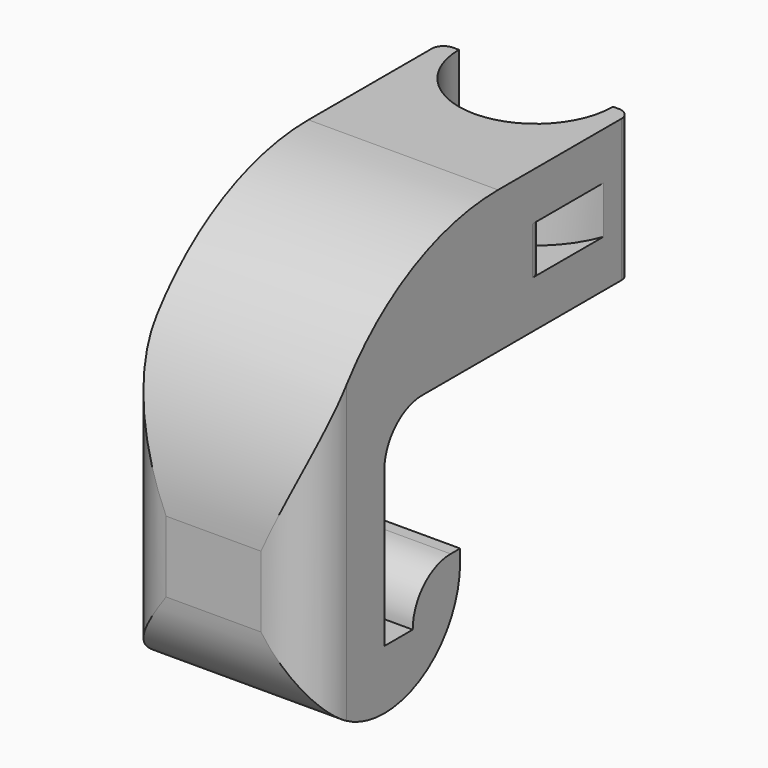
from build123d import *

# Parameters (mm, degrees)
F1_DEPTH     = 16
F2_R         = 7.99999
F3_R         = 20
F4_R         = 3.99999
F6_DEPTH     = 34.001
F8_DEPTH     = 4
F11_R        = 1
F12_T1_DEPTH = 33.00001


# Not quite as in the source:
# - a fillet or chamfer that OpenCascade refuses, or shapes differently, is made with other operations: its cross-section is extruded or revolved along the edge and cut away or added
# - a fillet or chamfer is up to 0.001 mm smaller than in the source, because OpenCascade refuses the exact size


with BuildPart() as f1:
    # F0 (on Right) → F1 (new body)
    with BuildSketch(Plane.YZ):
        Polygon((34, 34), (0, 34), (0, 0), (16, 0), (16, 9), (11, 9), (11, 5), (8, 5), (8, 22), (34, 22), align=None)
    extrude(amount=F1_DEPTH)

    # F2 (radius 8 in the source; OpenCascade refuses exactly that, so slightly less here)
    f2_edges = [f1.edges().sort_by_distance(p)[0] for p in [
        (8, 16, 0),
        (8, 0, 0),
    ]]
    fillet(f2_edges, radius=F2_R)

    # F3
    f3_edges = [f1.edges().sort_by_distance(p)[0] for p in [
        (8, 0, 34),
    ]]
    fillet(f3_edges, radius=F3_R)

    # F4 (radius 4 in the source; OpenCascade refuses exactly that, so slightly less here)
    f4_edges = [f1.edges().sort_by_distance(p)[0] for p in [
        (8, 8, 22),
        (8, 11, 9),
    ]]
    fillet(f4_edges, radius=F4_R)

    # F5 (on face) → F6 (cut, through all)
    with BuildSketch(Plane.XY.offset(34)):
        with BuildLine():
            ThreePointArc((1.5, 34), (8, 27.5), (14.5, 34))
            Line((14.5, 34), (1.5, 34))
        make_face()
    extrude(amount=-F6_DEPTH, mode=Mode.SUBTRACT)


with BuildPart() as f8:
    # F7 (on face) → F8 (new body)
    with BuildSketch(Plane.XY.offset(34)):
        with BuildLine():
            ThreePointArc((16, 31.1277186767), (8, 25.5), (0, 31.1277186767))
            Line((0, 31.1277186767), (0, 25.7386441791))
            ThreePointArc((0, 25.7386441791), (8, 22.5), (16, 25.7386441791))
            Line((16, 25.7386441791), (16, 31.1277186767))
        make_face()
    extrude(amount=F8_DEPTH)


with BuildPart() as f8_1:
    # F9: moved
    add(f8.part.moved(Location((0, 0, -8))))


with BuildPart() as f1_1:
    add(f1.part)

    # F10: cut F8
    add(f8_1.part, mode=Mode.SUBTRACT)

    # F11
    f11_edges = [f1_1.edges().sort_by_distance(p)[0] for p in [
        (16, 34, 28),
        (16, 25.738644, 28),
        (0, 34, 28),
        (0, 25.738644, 28),
    ]]
    fillet(f11_edges, radius=F11_R)

    # F12: fillet of radius 4 on 2 edges, made by hand

    # F12_s2 → F12_t1 (cut)
    with BuildSketch(Plane.XY.offset(-2.00001)):
        with BuildLine():
            ThreePointArc((12, 0), (14.8284271247, 1.1715728753), (16, 4))
            Line((16, 4), (16, 0))
            Line((16, 0), (12, 0))
        make_face()
        with BuildLine():
            ThreePointArc((0, 4), (1.1715728753, 1.1715728753), (4, 0))
            Line((4, 0), (0, 0))
            Line((0, 0), (0, 4))
        make_face()
    extrude(amount=F12_T1_DEPTH, mode=Mode.SUBTRACT)


solid = f1_1.part
